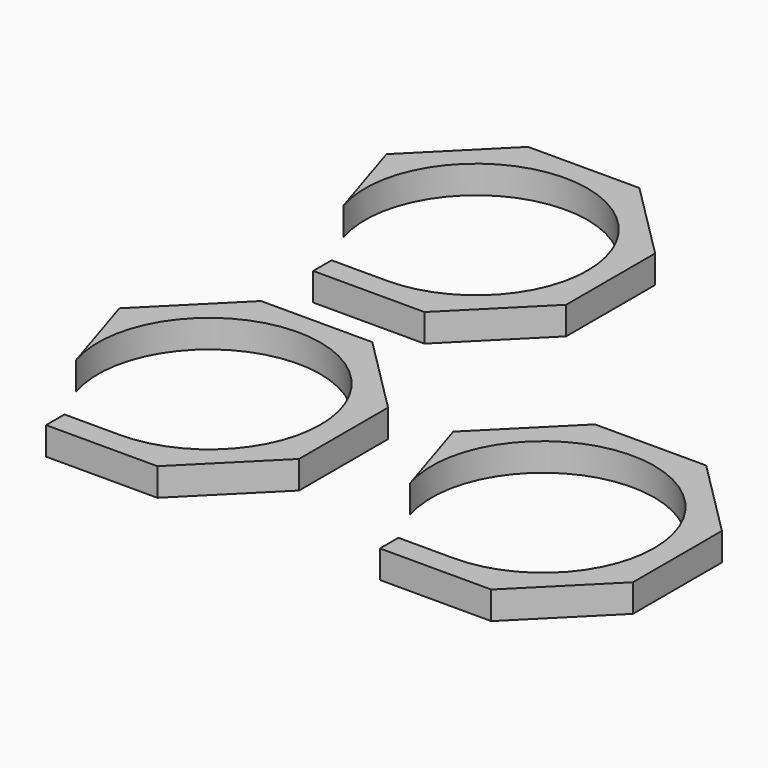
from build123d import *

# Parameters (mm, degrees)
F1_DEPTH = 3.175


# Not quite as in the source:
# - a length typed as a fraction of an inch, garbled in the dataset ("3 / 203.2 mm" for 3/8 in), is restored


with BuildPart() as f1:
    # F0 (on Top) → F1 (new body)
    with BuildSketch(Plane.XY):
        with BuildLine():
            Line((0, 2.6302561211), (0, 0))
            Line((0, 0), (12.7, 0))
            Line((12.7, 0), (15.24, 2.54))
            Line((15.24, 2.54), (21.6802561211, 8.9802561211))
            Line((21.6802561211, 8.9802561211), (21.6802561211, 21.6802561211))
            Line((21.6802561211, 21.6802561211), (19.1402561211, 24.2202561211))
            Line((19.1402561211, 24.2202561211), (12.7, 30.6605122421))
            Line((12.7, 30.6605122421), (0, 30.6605122421))
            Line((0, 30.6605122421), (-2.54, 28.1205122421))
            Line((-2.54, 28.1205122421), (-8.9802561211, 21.6802561211))
            Line((-8.9802561211, 21.6802561211), (-5.7581754145, 11.4985348197))
            ThreePointArc((-5.7581754145, 11.4985348197), (4.4114216245, 27.8814279342), (19.05, 15.3302561211))
            ThreePointArc((19.05, 15.3302561211), (15.3302561211, 6.35), (6.35, 2.6302561211))
            Line((6.35, 2.6302561211), (2.385919952, 2.6302561211))
            Line((2.385919952, 2.6302561211), (0, 2.6302561211))
        make_face()
    extrude(amount=F1_DEPTH)


with BuildPart() as f2_1:
    # F2: copy of F1
    add(f1.part.moved(Location((0, 38.1, 0))))


with BuildPart() as f3_1:
    # F3: copy of F1
    add(f1.part.moved(Location((38.1, 0, 0))))


solid = Compound([f1.part, f2_1.part, f3_1.part])
